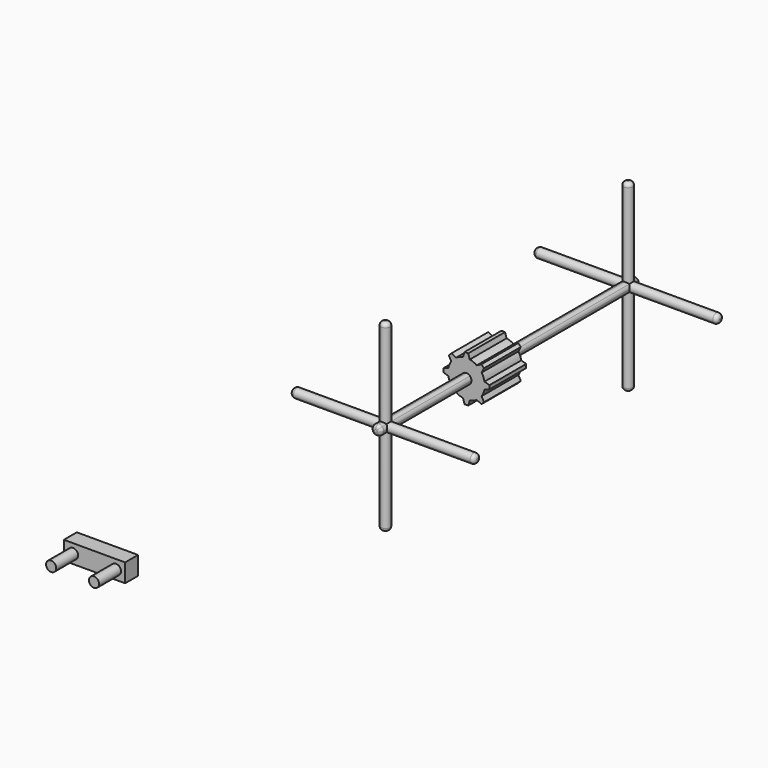
from build123d import *

# Parameters (mm, degrees)
F1_DEPTH       = 63.5
F2_R           = 6.985
F3_DEPTH       = 60.198
F2_W           = 84.582
F2_H           = 25.4
F4_DEPTH       = 22.352
F5_DEPTH       = 228.6
F5_DEPTH_BACK  = 219.964
F9_R           = 6.35
F10_DEPTH      = 127
F10_DEPTH_BACK = 127
F11_R          = 5.08
F13_R          = 6.35
F14_DEPTH      = 127
F14_DEPTH_BACK = 127
F15_R          = 5.08
F16_R          = 5.08
F18_R          = 6.35
F19_DEPTH      = 127
F19_DEPTH_BACK = 127
F20_R          = 6.35
F21_DEPTH      = 127
F21_DEPTH_BACK = 127
F22_R          = 5.08


# Not quite as in the source:
# - a feature of the source that left no trace in its solid (it failed there, or was rolled back) is left out


with BuildPart() as f1:
    # F0 (on Front) → F1 (new body)
    with BuildSketch(Plane.XZ):
        with BuildLine():
            Line((0, 31.75), (0, 25.4))
            ThreePointArc((0, 25.4), (2.348330872, 25.2912107681), (4.676545751, 24.9657749697))
            Line((4.676545751, 24.9657749697), (2.54, 31.75))
            Line((2.54, 31.75), (0, 31.75))
        make_face()
        with BuildLine():
            ThreePointArc((-4.676545751, 24.9657749697), (-2.348330872, 25.2912107681), (0, 25.4))
            Line((0, 25.4), (0, 31.75))
            Line((0, 31.75), (-2.54, 31.75))
            Line((-2.54, 31.75), (-4.676545751, 24.9657749697))
        make_face()
        with BuildLine():
            Line((-17.9605122421, 17.9605122421), (-4.9391408666, 4.9391408666))
            ThreePointArc((-4.9391408666, 4.9391408666), (-2.6730437751, 6.4532985346), (0, 6.985))
            Line((0, 6.985), (0, 25.4))
            ThreePointArc((0, 25.4), (-2.348330872, 25.2912107681), (-4.676545751, 24.9657749697))
            ThreePointArc((-4.676545751, 24.9657749697), (-9.6962229454, 23.4764405435), (-14.3038711395, 20.9895038156))
            ThreePointArc((-14.3038711395, 20.9895038156), (-16.2031264341, 19.5606414456), (-17.9605122421, 17.9605122421))
        make_face()
        with BuildLine():
            Line((-22.4506403027, 22.4506403027), (-17.9605122421, 17.9605122421))
            ThreePointArc((-17.9605122421, 17.9605122421), (-16.2031264341, 19.5606414456), (-14.3038711395, 20.9895038156))
            Line((-14.3038711395, 20.9895038156), (-20.6545890785, 24.2466915269))
            Line((-20.6545890785, 24.2466915269), (-22.4506403027, 22.4506403027))
        make_face()
        with BuildLine():
            ThreePointArc((-20.9895038156, 14.3038711395), (-19.5606414456, 16.2031264341), (-17.9605122421, 17.9605122421))
            Line((-17.9605122421, 17.9605122421), (-22.4506403027, 22.4506403027))
            Line((-22.4506403027, 22.4506403027), (-24.2466915269, 20.6545890785))
            Line((-24.2466915269, 20.6545890785), (-20.9895038156, 14.3038711395))
        make_face()
        with BuildLine():
            ThreePointArc((-4.9391408666, -4.9391408666), (-6.985, 0), (-4.9391408666, 4.9391408666))
            Line((-4.9391408666, 4.9391408666), (-17.9605122421, 17.9605122421))
            ThreePointArc((-17.9605122421, 17.9605122421), (-19.5606414456, 16.2031264341), (-20.9895038156, 14.3038711395))
            ThreePointArc((-20.9895038156, 14.3038711395), (-23.4764405435, 9.6962229454), (-24.9657749697, 4.676545751))
            ThreePointArc((-24.9657749697, 4.676545751), (-25.2912107681, 2.348330872), (-25.4, 0))
            ThreePointArc((-25.4, 0), (-25.2912107681, -2.348330872), (-24.9657749697, -4.676545751))
            ThreePointArc((-24.9657749697, -4.676545751), (-23.4764405435, -9.6962229454), (-20.9895038156, -14.3038711395))
            ThreePointArc((-20.9895038156, -14.3038711395), (-19.5606414456, -16.2031264341), (-17.9605122421, -17.9605122421))
            Line((-17.9605122421, -17.9605122421), (-4.9391408666, -4.9391408666))
        make_face()
        with BuildLine():
            Line((0, -25.4), (0, -6.985))
            ThreePointArc((0, -6.985), (-2.6730437751, -6.4532985346), (-4.9391408666, -4.9391408666))
            Line((-4.9391408666, -4.9391408666), (-17.9605122421, -17.9605122421))
            ThreePointArc((-17.9605122421, -17.9605122421), (-16.2031264341, -19.5606414456), (-14.3038711395, -20.9895038156))
            ThreePointArc((-14.3038711395, -20.9895038156), (-9.6962229454, -23.4764405435), (-4.676545751, -24.9657749697))
            ThreePointArc((-4.676545751, -24.9657749697), (-2.348330872, -25.2912107681), (0, -25.4))
        make_face()
        with BuildLine():
            ThreePointArc((4.9391408666, -4.9391408666), (2.6730437751, -6.4532985346), (0, -6.985))
            Line((0, -6.985), (0, -25.4))
            ThreePointArc((0, -25.4), (2.348330872, -25.2912107681), (4.676545751, -24.9657749697))
            ThreePointArc((4.676545751, -24.9657749697), (9.6962229454, -23.4764405435), (14.3038711395, -20.9895038156))
            ThreePointArc((14.3038711395, -20.9895038156), (16.2031264341, -19.5606414456), (17.9605122421, -17.9605122421))
            Line((17.9605122421, -17.9605122421), (4.9391408666, -4.9391408666))
        make_face()
        with BuildLine():
            Line((17.9605122421, 17.9605122421), (4.9391408666, 4.9391408666))
            ThreePointArc((4.9391408666, 4.9391408666), (6.4532985346, 2.6730437751), (6.985, 0))
            ThreePointArc((6.985, 0), (6.4532985346, -2.6730437751), (4.9391408666, -4.9391408666))
            Line((4.9391408666, -4.9391408666), (17.9605122421, -17.9605122421))
            ThreePointArc((17.9605122421, -17.9605122421), (19.5606414456, -16.2031264341), (20.9895038156, -14.3038711395))
            ThreePointArc((20.9895038156, -14.3038711395), (23.4764405435, -9.6962229454), (24.9657749697, -4.676545751))
            ThreePointArc((24.9657749697, -4.676545751), (25.2912107681, -2.348330872), (25.4, 0))
            ThreePointArc((25.4, 0), (25.2912107681, 2.348330872), (24.9657749697, 4.676545751))
            ThreePointArc((24.9657749697, 4.676545751), (23.4764405435, 9.6962229454), (20.9895038156, 14.3038711395))
            ThreePointArc((20.9895038156, 14.3038711395), (19.5606414456, 16.2031264341), (17.9605122421, 17.9605122421))
        make_face()
        with BuildLine():
            Line((0, 25.4), (0, 6.985))
            ThreePointArc((0, 6.985), (2.6730437751, 6.4532985346), (4.9391408666, 4.9391408666))
            Line((4.9391408666, 4.9391408666), (17.9605122421, 17.9605122421))
            ThreePointArc((17.9605122421, 17.9605122421), (16.2031264341, 19.5606414456), (14.3038711395, 20.9895038156))
            ThreePointArc((14.3038711395, 20.9895038156), (9.6962229454, 23.4764405435), (4.676545751, 24.9657749697))
            ThreePointArc((4.676545751, 24.9657749697), (2.348330872, 25.2912107681), (0, 25.4))
        make_face()
        with BuildLine():
            Line((22.4506403027, 22.4506403027), (17.9605122421, 17.9605122421))
            ThreePointArc((17.9605122421, 17.9605122421), (19.5606414456, 16.2031264341), (20.9895038156, 14.3038711395))
            Line((20.9895038156, 14.3038711395), (24.2466915269, 20.6545890785))
            Line((24.2466915269, 20.6545890785), (22.4506403027, 22.4506403027))
        make_face()
        with BuildLine():
            ThreePointArc((14.3038711395, 20.9895038156), (16.2031264341, 19.5606414456), (17.9605122421, 17.9605122421))
            Line((17.9605122421, 17.9605122421), (22.4506403027, 22.4506403027))
            Line((22.4506403027, 22.4506403027), (20.6545890785, 24.2466915269))
            Line((20.6545890785, 24.2466915269), (14.3038711395, 20.9895038156))
        make_face()
        with BuildLine():
            Line((31.75, 2.54), (24.9657749697, 4.676545751))
            ThreePointArc((24.9657749697, 4.676545751), (25.2912107681, 2.348330872), (25.4, 0))
            Line((25.4, 0), (31.75, 0))
            Line((31.75, 0), (31.75, 2.54))
        make_face()
        with BuildLine():
            ThreePointArc((25.4, 0), (25.2912107681, -2.348330872), (24.9657749697, -4.676545751))
            Line((24.9657749697, -4.676545751), (31.75, -2.54))
            Line((31.75, -2.54), (31.75, 0))
            Line((31.75, 0), (25.4, 0))
        make_face()
        with BuildLine():
            ThreePointArc((20.9895038156, -14.3038711395), (19.5606414456, -16.2031264341), (17.9605122421, -17.9605122421))
            Line((17.9605122421, -17.9605122421), (22.4506403027, -22.4506403027))
            Line((22.4506403027, -22.4506403027), (24.2466915269, -20.6545890785))
            Line((24.2466915269, -20.6545890785), (20.9895038156, -14.3038711395))
        make_face()
        with BuildLine():
            Line((22.4506403027, -22.4506403027), (17.9605122421, -17.9605122421))
            ThreePointArc((17.9605122421, -17.9605122421), (16.2031264341, -19.5606414456), (14.3038711395, -20.9895038156))
            Line((14.3038711395, -20.9895038156), (20.6545890785, -24.2466915269))
            Line((20.6545890785, -24.2466915269), (22.4506403027, -22.4506403027))
        make_face()
        with BuildLine():
            ThreePointArc((4.676545751, -24.9657749697), (2.348330872, -25.2912107681), (0, -25.4))
            Line((0, -25.4), (0, -31.75))
            Line((0, -31.75), (2.54, -31.75))
            Line((2.54, -31.75), (4.676545751, -24.9657749697))
        make_face()
        with BuildLine():
            Line((0, -31.75), (0, -25.4))
            ThreePointArc((0, -25.4), (-2.348330872, -25.2912107681), (-4.676545751, -24.9657749697))
            Line((-4.676545751, -24.9657749697), (-2.54, -31.75))
            Line((-2.54, -31.75), (0, -31.75))
        make_face()
        with BuildLine():
            ThreePointArc((-14.3038711395, -20.9895038156), (-16.2031264341, -19.5606414456), (-17.9605122421, -17.9605122421))
            Line((-17.9605122421, -17.9605122421), (-22.4506403027, -22.4506403027))
            Line((-22.4506403027, -22.4506403027), (-20.6545890785, -24.2466915269))
            Line((-20.6545890785, -24.2466915269), (-14.3038711395, -20.9895038156))
        make_face()
        with BuildLine():
            Line((-22.4506403027, -22.4506403027), (-17.9605122421, -17.9605122421))
            ThreePointArc((-17.9605122421, -17.9605122421), (-19.5606414456, -16.2031264341), (-20.9895038156, -14.3038711395))
            Line((-20.9895038156, -14.3038711395), (-24.2466915269, -20.6545890785))
            Line((-24.2466915269, -20.6545890785), (-22.4506403027, -22.4506403027))
        make_face()
        with BuildLine():
            ThreePointArc((-25.4, 0), (-25.2912107681, 2.348330872), (-24.9657749697, 4.676545751))
            Line((-24.9657749697, 4.676545751), (-31.75, 2.54))
            Line((-31.75, 2.54), (-31.75, 0))
            Line((-31.75, 0), (-31.75, -2.54))
            Line((-31.75, -2.54), (-24.9657749697, -4.676545751))
            ThreePointArc((-24.9657749697, -4.676545751), (-25.2912107681, -2.348330872), (-25.4, 0))
        make_face()
    extrude(amount=F1_DEPTH)

    # F0 (on Front) → F5 (join, two sides)
    with BuildSketch(Plane.XZ) as f5_sk:
        with BuildLine():
            Line((4.9391408666, -4.9391408666), (0, 0))
            Line((0, 0), (0, -6.985))
            ThreePointArc((0, -6.985), (2.6730437751, -6.4532985346), (4.9391408666, -4.9391408666))
        make_face()
        with BuildLine():
            Line((0, -6.985), (0, 0))
            Line((0, 0), (-4.9391408666, -4.9391408666))
            ThreePointArc((-4.9391408666, -4.9391408666), (-2.6730437751, -6.4532985346), (0, -6.985))
        make_face()
        with BuildLine():
            Line((-4.9391408666, -4.9391408666), (0, 0))
            Line((0, 0), (-4.9391408666, 4.9391408666))
            ThreePointArc((-4.9391408666, 4.9391408666), (-6.985, 0), (-4.9391408666, -4.9391408666))
        make_face()
        with BuildLine():
            Line((-4.9391408666, 4.9391408666), (0, 0))
            Line((0, 0), (0, 6.985))
            ThreePointArc((0, 6.985), (-2.6730437751, 6.4532985346), (-4.9391408666, 4.9391408666))
        make_face()
        with BuildLine():
            Line((0, 6.985), (0, 0))
            Line((0, 0), (4.9391408666, 4.9391408666))
            ThreePointArc((4.9391408666, 4.9391408666), (2.6730437751, 6.4532985346), (0, 6.985))
        make_face()
        with BuildLine():
            Line((4.9391408666, 4.9391408666), (0, 0))
            Line((0, 0), (4.9391408666, -4.9391408666))
            ThreePointArc((4.9391408666, -4.9391408666), (6.4532985346, -2.6730437751), (6.985, 0))
            ThreePointArc((6.985, 0), (6.4532985346, 2.6730437751), (4.9391408666, 4.9391408666))
        make_face()
    extrude(amount=-F5_DEPTH)
    extrude(f5_sk.sketch, amount=F5_DEPTH_BACK)


with BuildPart() as f3:
    # F2 (on Front) → F3 (new body)
    with BuildSketch(Plane.XZ):
        with Locations((-19.2150007933, 47.4165305495)):
            Circle(F2_R)
    extrude(amount=F3_DEPTH)


with BuildPart() as f3b:
    # F2 (on Front) → F3, piece 2 (new body)
    with BuildSketch(Plane.XZ):
        with Locations((39.9669992067, 47.4165305495)):
            Circle(F2_R)
    extrude(amount=F3_DEPTH)


with BuildPart() as f4:
    # F2 (on Front) → F4 (new body)
    with BuildSketch(Plane.XZ):
        with Locations((10.3759992067, 47.4165305495)):
            Rectangle(F2_W, F2_H)
        with Locations((-19.2150007933, 47.4165305495)):
            Circle(F2_R, mode=Mode.SUBTRACT)
        with Locations((39.9669992067, 47.4165305495)):
            Circle(F2_R, mode=Mode.SUBTRACT)
    extrude(amount=F4_DEPTH)


with BuildPart() as f1_1:
    # F6: moved
    add(f1.part.moved(Location((0, -132.08, 0))))


with BuildPart() as f1_2:
    # F8: moved
    add(f1_1.part.moved(Location((0, -83.566, 0))))

    # F9 (on Right) → F10 (join, two sides)
    with BuildSketch(Plane.YZ) as f10_sk:
        Circle(F9_R)
    extrude(amount=F10_DEPTH)
    extrude(f10_sk.sketch, amount=-F10_DEPTH_BACK)

    # F11
    f11_edges = [f1_2.edges().sort_by_distance(p)[0] for p in [
        (-127, -6.35, 0),
        (127, -6.35, 0),
    ]]
    fillet(f11_edges, radius=F11_R)

    # F13 (on Top) → F14 (join, two sides)
    with BuildSketch(Plane.XY) as f14_sk:
        Circle(F13_R)
    extrude(amount=F14_DEPTH)
    extrude(f14_sk.sketch, amount=-F14_DEPTH_BACK)

    # F15
    f15_edges = [f1_2.edges().sort_by_distance(p)[0] for p in [
        (-6.35, 0, 127),
        (-6.35, 0, -127),
    ]]
    fillet(f15_edges, radius=F15_R)

    # F16
    f16_edges = [f1_2.edges().sort_by_distance(p)[0] for p in [
        (-4.939141, -435.61, 4.939141),
    ]]
    fillet(f16_edges, radius=F16_R)


with BuildPart() as f3_1:
    # F12: moved
    add(f3.part.moved(Location((0, -492.76, 0))))


with BuildPart() as f4_1:
    # F12: moved
    add(f4.part.moved(Location((0, -492.76, 0))))


with BuildPart() as f3b_1:
    # F12: moved
    add(f3b.part.moved(Location((0, -492.76, 0))))


with BuildPart() as f1_3:
    # F17: moved
    add(f1_2.part.moved(Location((0, 418.846, 0))))

    # F18 (on Top) → F19 (join, two sides)
    with BuildSketch(Plane.XY) as f19_sk:
        Circle(F18_R)
    extrude(amount=F19_DEPTH)
    extrude(f19_sk.sketch, amount=-F19_DEPTH_BACK)

    # F20 (on Right) → F21 (join, two sides)
    with BuildSketch(Plane.YZ) as f21_sk:
        Circle(F20_R)
    extrude(amount=F21_DEPTH)
    extrude(f21_sk.sketch, amount=-F21_DEPTH_BACK)

    # F22
    f22_edges = [f1_3.edges().sort_by_distance(p)[0] for p in [
        (127, -6.35, 0),
        (-6.35, 0, -127),
        (-127, -6.35, 0),
        (-6.35, 0, 127),
        (-4.939141, 431.8, 4.939141),
    ]]
    fillet(f22_edges, radius=F22_R)


solid = Compound([f3_1.part, f4_1.part, f3b_1.part, f1_3.part])
